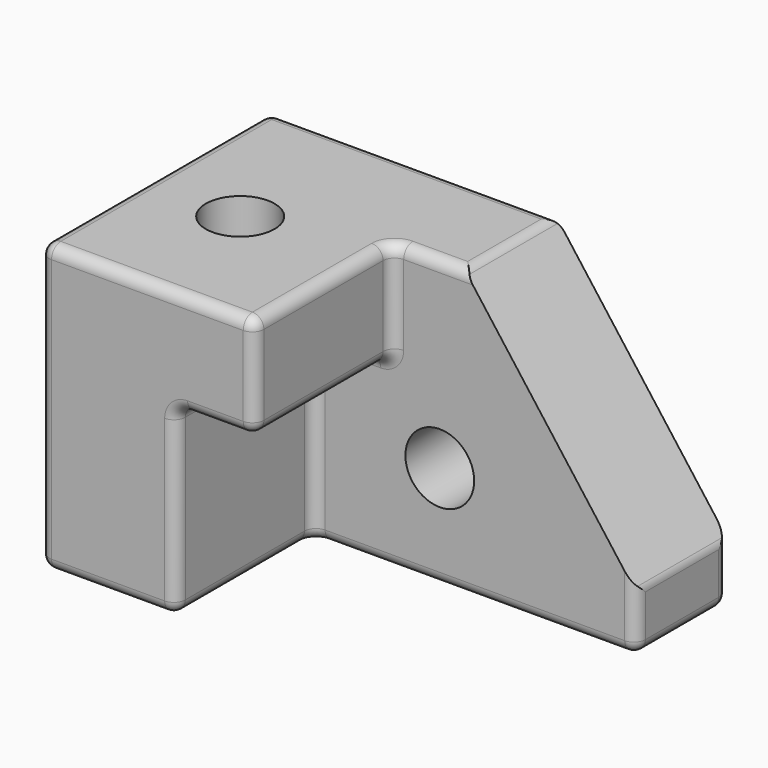
from build123d import *

# Parameters (mm, degrees)
F0_W     = 203.2
F0_H     = 127
F1_DEPTH = 127
F3_DEPTH = 76.2
F4_SIZE2 = 101.6
F4_SIZE  = 76.2
F5_R     = 5.08
F6_R     = 15.24
F7_DEPTH = 50.8
F8_R     = 15.24
F9_DEPTH = 127


with BuildPart() as f1:
    # F0 (on Front) → F1 (new body)
    with BuildSketch(Plane.XZ):
        with Locations((41.3226257026, 20.5530026861)):
            Rectangle(F0_W, F0_H)
    extrude(amount=F1_DEPTH)

    # F2 (on face) → F3 (cut)
    with BuildSketch(Plane.XZ.offset(127)):
        Polygon((142.9226257026, 84.0530026861), (34.8217822611, 84.0530026861), (34.8217822611, 38.4303182364), (0, 38.4303182364), (0, -42.9469973139), (142.9226257026, -42.9469973139), align=None)
    extrude(amount=-F3_DEPTH, mode=Mode.SUBTRACT)

    # F4
    f4_edges = [f1.edges().sort_by_distance(p)[0] for p in [
        (142.922626, -25.4, 84.053003),
    ]]
    f4_side = f1.faces().sort_by_distance((19.028994, -51.591204, 84.053003))[0]
    chamfer(f4_edges, length=F4_SIZE, length2=F4_SIZE2, reference=f4_side)

    # F5
    f5_edges = [f1.edges().sort_by_distance(p)[0] for p in [
        (34.821782, -88.9, 84.053003),
        (0, -127, -2.25834),
        (50.772204, -50.8, 84.053003),
        (34.821782, -50.8, 61.24166),
        (34.821782, -127, 61.24166),
        (17.410891, -127, 38.430318),
        (-30.138687, -127, -42.946997),
        (-60.277374, -127, 20.553003),
        (-12.727796, -127, 84.053003),
        (3.222626, 0, 84.053003),
        (66.722626, -25.4, 84.053003),
        (-60.277374, -63.5, 84.053003),
        (0, -50.8, -2.25834),
        (0, -88.9, 38.430318),
        (0, -88.9, -42.946997),
        (142.922626, 0, -30.246997),
        (142.922626, -25.4, -17.546997),
        (142.922626, -25.4, -42.946997),
        (142.922626, -50.8, -30.246997),
        (41.322626, 0, -42.946997),
        (-60.277374, 0, 20.553003),
        (-60.277374, -63.5, -42.946997),
        (34.821782, -88.9, 38.430318),
        (17.410891, -50.8, 38.430318),
        (71.461313, -50.8, -42.946997),
    ]]
    fillet(f5_edges, radius=F5_R)

    # F6 (on face) → F7 (cut, through all)
    with BuildSketch(Plane.XZ.offset(50.8)):
        with Locations((55.88, 2.7730026861)):
            Circle(F6_R)
    extrude(amount=-F7_DEPTH, mode=Mode.SUBTRACT)

    # F8 (on face) → F9 (cut, through all)
    with BuildSketch(Plane.XY.offset(84.0530026861)):
        with Locations((-18.4064079076, -68.5097798705)):
            Circle(F8_R)
    extrude(amount=-F9_DEPTH, mode=Mode.SUBTRACT)


solid = f1.part
